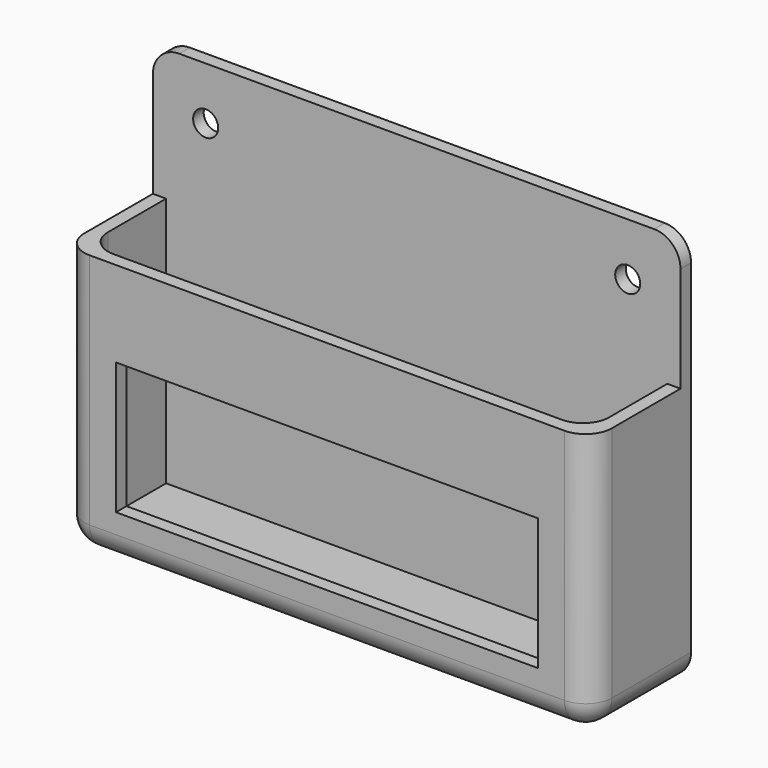
from build123d import *

# Parameters (mm, degrees)
F0_W      = 101.6
F0_H      = 76.2
F1_DEPTH  = 2.54
F2_W      = 101.6
F2_H      = 50.8
F3_DEPTH  = 21.59
F4_R      = 5.08
F5_W      = 96.52
F5_H      = 19.05
F6_DEPTH  = 48.26
F7_R      = 5.08
F8_R      = 5.08
F9_R      = 5.08
F11_W     = 81.28
F11_H     = 25.4
F12_DEPTH = 21.59
F13_R     = 2.413
F14_DEPTH = 2.541


# Not quite as in the source:
# - a feature of the source that left no trace in its solid (it failed there, or was rolled back) is left out


with BuildPart() as f1:
    # F0 (on Front) → F1 (new body)
    with BuildSketch(Plane.XZ):
        with Locations((50.8, 38.1)):
            Rectangle(F0_W, F0_H)
    extrude(amount=F1_DEPTH)

    # F2 (on face) → F3 (join)
    with BuildSketch(Plane.XZ.offset(2.54)):
        with Locations((50.8, 25.4)):
            Rectangle(F2_W, F2_H)
    extrude(amount=F3_DEPTH)

    # F4
    f4_edges = [f1.edges().sort_by_distance(p)[0] for p in [
        (101.6, -1.27, 76.2),
        (101.6, -12.065, 0),
        (0, -12.065, 0),
        (0, -1.27, 76.2),
    ]]
    fillet(f4_edges, radius=F4_R)

    # F5 (on face) → F6 (cut)
    with BuildSketch(Plane.XY.offset(50.8)):
        with Locations((50.8, -12.065)):
            Rectangle(F5_W, F5_H)
    extrude(amount=-F6_DEPTH, mode=Mode.SUBTRACT)

    # F7
    f7_edges = [f1.edges().sort_by_distance(p)[0] for p in [
        (101.6, -24.13, 27.94),
    ]]
    fillet(f7_edges, radius=F7_R)

    # F8
    f8_edges = [f1.edges().sort_by_distance(p)[0] for p in [
        (99.06, -21.59, 26.67),
    ]]
    fillet(f8_edges, radius=F8_R)

    # F9
    f9_edges = [f1.edges().sort_by_distance(p)[0] for p in [
        (2.54, -21.59, 26.67),
    ]]
    fillet(f9_edges, radius=F9_R)

    # F11 (on face) → F12 (cut, through all)
    with BuildSketch(Plane.XZ.offset(24.13)):
        with Locations((50.8, 21.59)):
            Rectangle(F11_W, F11_H)
    extrude(amount=-F12_DEPTH, mode=Mode.SUBTRACT)

    # F13 (on face) → F14 (cut, through all)
    with BuildSketch(Plane.XZ.offset(2.54)):
        with Locations((91.44, 66.04)):
            Circle(F13_R)
        with Locations((10.16, 66.04)):
            Circle(F13_R)
    extrude(amount=-F14_DEPTH, mode=Mode.SUBTRACT)


solid = f1.part
